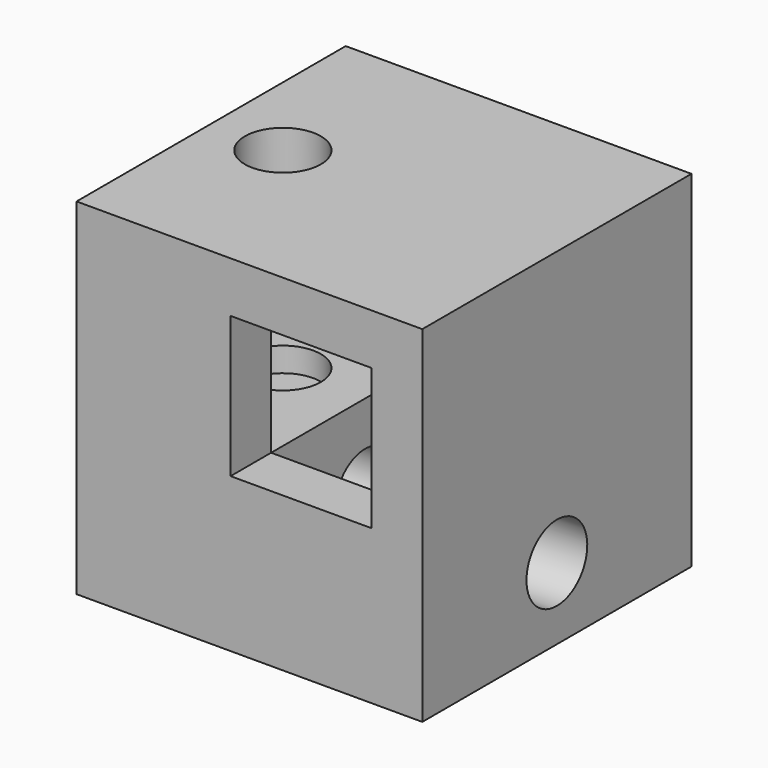
from build123d import *

# Parameters (mm, degrees)
F0_W     = 21.6662
F0_H     = 21.6662
F1_DEPTH = 3.175
F2_W     = 18.4912
F2_H     = 3.175
F2_W_2   = 9.652
F2_H_2   = 9.652
F3_DEPTH = 14.732
F5_DEPTH = 13.5382
F7_DEPTH = 25.4
F9_DEPTH = 3.175


# Not quite as in the source:
# - a length typed as a fraction of an inch, garbled in the dataset ("3 / 203.2 mm" for 3/8 in), is restored


with BuildPart() as f1:
    # F0 (on Front) → F1 (new body)
    with BuildSketch(Plane.XZ):
        with Locations((-21.4400560975, -33.0820980474)):
            Rectangle(F0_W, F0_H)
    extrude(amount=F1_DEPTH)

    # F2 (on face) → F3 (join)
    with BuildSketch(Plane.XZ.offset(3.175)):
        with Locations((-23.0275560975, -23.8364980474)):
            Rectangle(F2_W, F2_H)
        Polygon((-13.7819560975, -22.2489980474), (-13.7819560975, -25.4239980474), (-13.7819560975, -43.9151980474), (-10.6069560975, -43.9151980474), (-10.6069560975, -22.2489980474), align=None)
        with Locations((-27.4471560975, -39.0891980474)):
            Rectangle(F2_W_2, F2_H_2)
    extrude(amount=F3_DEPTH)

    # F4 (on face) → F5 (cut)
    with BuildSketch(Plane.XY.offset(-22.2489980474)):
        with BuildLine():
            ThreePointArc((-25.3961060975, -10.541), (-27.7773560975, -8.15975), (-30.1586060975, -10.541))
            ThreePointArc((-30.1586060975, -10.541), (-27.7773560975, -12.92225), (-25.3961060975, -10.541))
        make_face()
    extrude(amount=-F5_DEPTH, mode=Mode.SUBTRACT)

    # F6 (on face) → F7 (cut)
    with BuildSketch(Plane.YZ.offset(-10.6069560975)):
        with BuildLine():
            ThreePointArc((-8.15975, -39.4193980474), (-12.2247980227, -37.7356000247), (-10.541, -41.8006480474))
            ThreePointArc((-10.541, -41.8006480474), (-8.8572019773, -41.1031960701), (-8.15975, -39.4193980474))
        make_face()
    extrude(amount=-F7_DEPTH, mode=Mode.SUBTRACT)

    # F8 (on face) → F9 (join)
    with BuildSketch(Plane.XZ.offset(17.907)):
        Polygon((-10.6069560975, -43.9151980474), (-10.6069560975, -22.2489980474), (-32.2731560975, -22.2489980474), (-32.2731560975, -25.4239980474), (-22.6211560975, -25.4239980474), (-13.7819560975, -25.4239980474), (-13.7819560975, -34.2631980474), (-13.7819560975, -43.9151980474), align=None)
        Polygon((-22.6211560975, -25.4239980474), (-32.2731560975, -25.4239980474), (-32.2731560975, -43.9151980474), (-13.7819560975, -43.9151980474), (-13.7819560975, -34.2631980474), (-22.6211560975, -34.2631980474), align=None)
    extrude(amount=F9_DEPTH)


solid = f1.part
